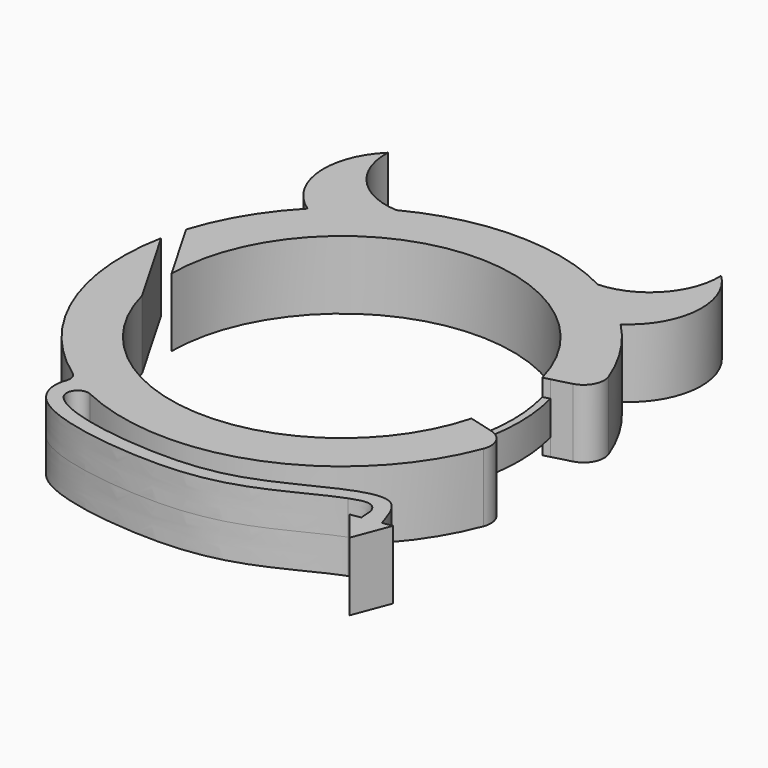
from build123d import *

# Parameters (mm, degrees)
F1_DEPTH = 2.5
F2_DEPTH = 1.25
F3_R     = 1.5
F4_DEPTH = 2.5
F5_R     = 0.8


# Not quite as in the source:
# - ends of sketch curves that miss each other by under 0.0002 mm in the source are joined
# - the dataset's text gives a spline's control points without its knots; the knots are read off the source's solid


with BuildPart() as f1:
    # F0 (on Top) → F1 (new body, symmetric)
    with BuildSketch(Plane.XY):
        with BuildLine():
            ThreePointArc((-12.4997921931, 0.0720772397), (-1.5958401687, 12.3977132632), (12.0740728286, 3.2352380638))
            Line((12.0740728286, 3.2352380638), (12.5570357418, 3.3646475863))
            Line((12.5570357418, 3.3646475863), (15.4548132206, 4.1411047216))
            ThreePointArc((15.4548132206, 4.1411047216), (13.9025925761, 7.9194646071), (11.4442382915, 11.1816550621))
            ThreePointArc((11.4442382915, 11.1816550621), (9.5223590052, 12.8578644796), (7.3585783975, 14.2074390362))
            ThreePointArc((7.3585783975, 14.2074390362), (0, 16), (-7.3585783975, 14.2074390362))
            ThreePointArc((-7.3585783975, 14.2074390362), (-9.5223590052, 12.8578644796), (-11.4442382915, 11.1816550621))
            ThreePointArc((-11.4442382915, 11.1816550621), (-13.7194334915, 8.2326875729), (-15.2511574536, 4.8375816609))
            Line((-15.2511574536, 4.8375816609), (-12.4997921931, 0.0720772397))
        make_face()
        with BuildLine():
            ThreePointArc((-12.1797463165, 19.4514751915), (-13.7905135345, 15.1405977877), (-11.4442382915, 11.1816550621))
            ThreePointArc((-11.4442382915, 11.1816550621), (-9.5223590052, 12.8578644796), (-7.3585783975, 14.2074390362))
            ThreePointArc((-7.3585783975, 14.2074390362), (-10.8510358044, 15.8348237051), (-12.1797463165, 19.4514751915))
        make_face()
        with BuildLine():
            ThreePointArc((7.3585783975, 14.2074390362), (9.5223590052, 12.8578644796), (11.4442382915, 11.1816550621))
            ThreePointArc((11.4442382915, 11.1816550621), (13.7905135345, 15.1405977877), (12.1797463165, 19.4514751915))
            ThreePointArc((12.1797463165, 19.4514751915), (10.8510358044, 15.8348237051), (7.3585783975, 14.2074390362))
        make_face()
    extrude(amount=F1_DEPTH, both=True)



with BuildPart() as f1b:
    # F0 (on Top) → F1, piece 2 (new body, symmetric)
    with BuildSketch(Plane.XY):
        with BuildLine():
            Line((12.5570357418, -3.3646475863), (12.0740728286, -3.2352380638))
            ThreePointArc((12.0740728286, -3.2352380638), (-0.0662546533, -12.4998244116), (-12.1076898624, -3.107063919))
            Line((-12.1076898624, -3.107063919), (-15.6954182424, 3.107063919))
            ThreePointArc((-15.6954182424, 3.107063919), (-14.7280011146, -6.2518783712), (-8.6675896137, -13.4488992222))
            ThreePointArc((-8.6675896137, -13.4488992222), (-8.2430782578, -13.7131929483), (-7.8105150545, -13.9640916133))
            ThreePointArc((-7.8105150545, -13.9640916133), (6.2234710156, -14.740027426), (15.4548132206, -4.1411047216))
            Line((15.4548132206, -4.1411047216), (12.5570357418, -3.3646475863))
        make_face()
        with BuildLine():
            ThreePointArc((-7.8105150545, -13.9640916133), (-8.2430782578, -13.7131929483), (-8.6675896137, -13.4488992222))
            add(Edge.make_bspline(
                [(-8.6675896137, -13.4488992222), (-8.797764652, -13.6654585416), (-9.0152035334, -14.1398334202), (-9.1106271715, -14.8441369677), (-9.019453346, -15.4402355626), (-8.8577356601, -15.8805060204), (-8.606122993, -16.2902925258), (-8.2704537018, -16.6576498092), (-7.8814651413, -16.9636616263), (-7.3119803281, -17.3112660682), (-6.5035804076, -17.6685037974), (-5.3935521754, -18.017298843), (-4.1682718306, -18.2991057591), (-2.8605703232, -18.5187890962), (-1.5067823109, -18.6776427369), (-0.1448831469, -18.7755760581), (1.1866806091, -18.811715906), (2.4507043421, -18.7843156845), (3.6107265904, -18.6908897447), (4.6838851631, -18.5342313543), (6.0200948318, -18.2454330252), (7.2429524692, -17.8461078269), (8.4161128097, -17.360744608), (9.2884492722, -16.9607714916), (10.1788682347, -16.5256334939), (11.0786073367, -16.0789478737), (11.9458288341, -15.6684730299), (12.4853133495, -15.4419413174), (12.735188331, -15.3475727395)],
                knots=[0, 0, 0, 0, 0.03125, 0.0625, 0.078125, 0.09375, 0.109375, 0.125, 0.140625, 0.15625, 0.1875, 0.21875, 0.25, 0.28125, 0.3125, 0.34375, 0.375, 0.40625, 0.4375, 0.46875, 0.5, 0.5625, 0.59375, 0.625, 0.65625, 0.6875, 0.71875, 0.7488919453, 0.7488919453, 0.7488919453, 0.7488919453], degree=3))
            add(Edge.make_bspline(
                [(12.735188331, -15.3475727395), (13.0962225988, -15.2263056252), (14.0987647195, -14.8169575852), (14.8734039357, -15.6872366698), (14.744015393, -16.4765788546), (14.8353977892, -16.7206706709)],
                knots=[0, 0, 0, 0, 0.3705867105, 0.6816060498, 1, 1, 1, 1], degree=3))
            Line((14.8353977892, -16.7206706709), (16.1413460697, -16.5104982377))
            add(Edge.make_bspline(
                [(-7.8105150545, -13.9640916133), (-8.1627060189, -14.5499968418), (-8.3932358627, -16.9546025127), (3.0722998689, -18.5185205906), (8.7653437405, -16.2477641355), (15.1718434378, -12.7619138207), (15.864960823, -15.7065625014), (16.1413460697, -16.5104982377)],
                knots=[0, 0, 0, 0, 0.1227588113, 0.403467238, 0.6434540436, 0.8535085955, 1, 1, 1, 1], degree=3))
        make_face()
        Polygon((16.8711597868, -16.3930458647), (16.1413460697, -16.5104982377), (14.8353977892, -16.7206706709), (14.0320850357, -16.8499515915), (15.8481355757, -19.0853122622), align=None)
    extrude(amount=F1_DEPTH, both=True)


with BuildPart() as f1_1:
    add(f1.part)

    add(f1b.part)  # F2 merges F1b
    # F0 (on Top) → F2 (join, symmetric)
    with BuildSketch(Plane.XY):
        with BuildLine():
            ThreePointArc((12.0740728286, 3.2352380638), (12.3930607672, 1.6315774028), (12.5, 0))
            ThreePointArc((12.5, 0), (12.3930607672, -1.6315774028), (12.0740728286, -3.2352380638))
            Line((12.0740728286, -3.2352380638), (12.5570357418, -3.3646475863))
            ThreePointArc((12.5570357418, -3.3646475863), (13, 0), (12.5570357418, 3.3646475863))
            Line((12.5570357418, 3.3646475863), (12.0740728286, 3.2352380638))
        make_face()
    extrude(amount=F2_DEPTH, both=True)

    # F3
    f3_edges = [f1_1.edges().sort_by_distance(p)[0] for p in [
        (15.454813, -4.141105, 0),
        (15.454813, 4.141105, 0),
    ]]
    fillet(f3_edges, radius=F3_R)

    # F0 (on Top) → F4 (cut, symmetric)
    with BuildSketch(Plane.XY):
        with BuildLine():
            ThreePointArc((12.0740728286, -3.2352380638), (12.3930607672, -1.6315774028), (12.5, 0))
            ThreePointArc((12.5, 0), (12.3930607672, 1.6315774028), (12.0740728286, 3.2352380638))
            ThreePointArc((12.0740728286, 3.2352380638), (-1.5958401687, 12.3977132632), (-12.4997921931, 0.0720772397))
            ThreePointArc((-12.4997921931, 0.0720772397), (-12.4059976586, -1.5301052563), (-12.1076898624, -3.107063919))
            ThreePointArc((-12.1076898624, -3.107063919), (-0.0662546533, -12.4998244116), (12.0740728286, -3.2352380638))
        make_face()
    extrude(amount=F4_DEPTH, both=True, mode=Mode.SUBTRACT)

    # F5
    f5_edges = [f1_1.edges().sort_by_distance(p)[0] for p in [
        (-7.810515, -13.964092, 1.25),
        (-7.810515, -13.964092, -1.25),
        (-8.66759, -13.448899, 1.25),
        (-8.66759, -13.448899, -1.25),
    ]]
    fillet(f5_edges, radius=F5_R)


solid = f1_1.part
